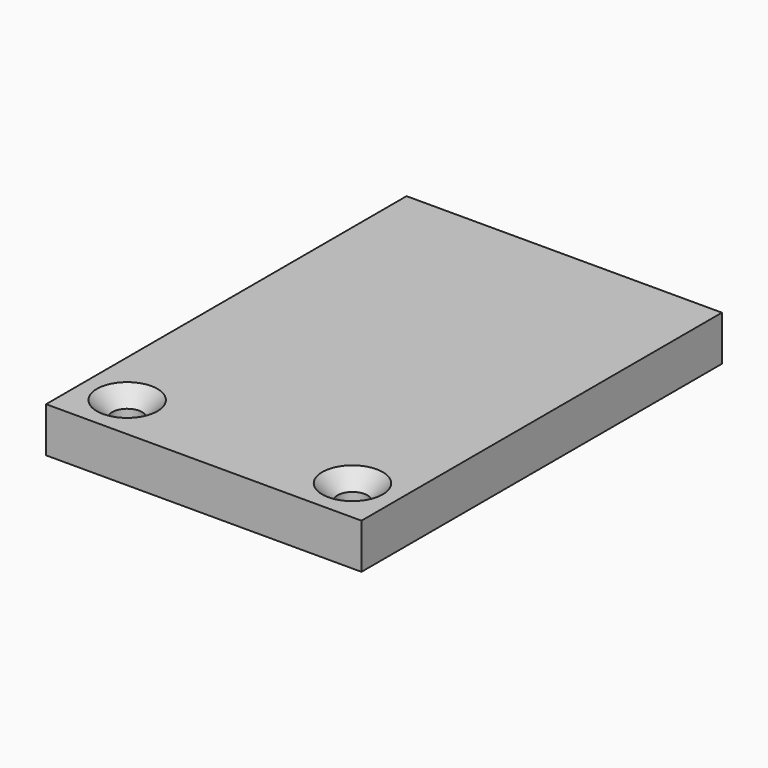
from build123d import *

# Parameters (mm, degrees)
F0_W           = 70
F0_H           = 100
F1_DEPTH       = 10
F3_D           = 6.6
F3_CSINK_D     = 13.44
F3_CSINK_ANGLE = 90


# Not quite as in the source:
# - a pattern or mirror of a feature is missing from the dataset's text; its kind, count and spacing are read off the source's solid


with BuildPart() as f1:
    # F0 (on Top) → F1 (new body)
    with BuildSketch(Plane.XY):
        with Locations((0, 40)):
            Rectangle(F0_W, F0_H)
    extrude(amount=F1_DEPTH)

    # F3 (through all)
    with Locations(Plane.XY.offset(10)):
        with Locations((-25, 0)):
            f3 = CounterSinkHole(F3_D / 2, F3_CSINK_D / 2, counter_sink_angle=F3_CSINK_ANGLE)

    # F3_copies: F3 across plane
    add(f3.mirror(Plane(origin=(0, 0, 0), x_dir=(0, 0, 1), z_dir=(1, 0, 0))), mode=Mode.SUBTRACT)


solid = f1.part
